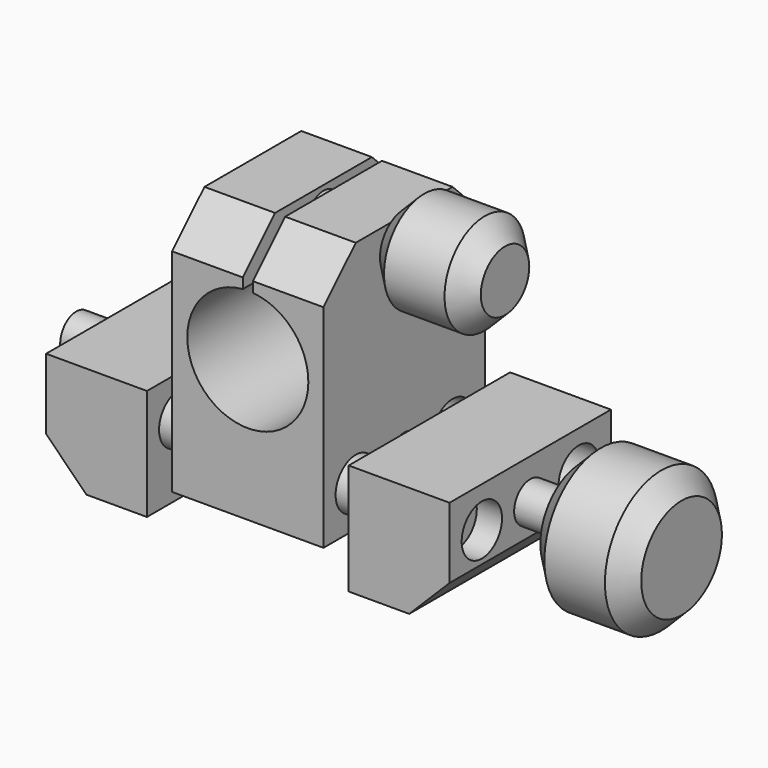
from build123d import *

# Parameters (mm, degrees)
F1_DEPTH      = 20
F2_R          = 2.5
F2_R_2        = 2
F3_DEPTH      = 7.501
F3_DEPTH_BACK = 7.501
F4_DEPTH      = 17.5
F5_START      = 10
F2_W          = 20
F2_H          = 11
F5_DEPTH      = 10
F6_START      = -10
F6_DEPTH      = 10
F7_D          = 3.3
F8_SIZE       = 4
F8_2_SIZE     = 4
F9_SIZE       = 4
F10_DEPTH     = 25
F11_R         = 7
F12_DEPTH     = 10
F14_D         = 3.3
F14_DEPTH     = 7.501
F15_D         = 4.2
F15_DEPTH     = 7.501
F16_SIZE      = 0.5
F17_R         = 2
F18_DEPTH     = 15
F19_R         = 5
F20_DEPTH     = 10
F21_SIZE      = 2
F21_2_SIZE    = 2
F22_SIZE      = 1


with BuildPart() as f1:
    # F0 (on Front) → F1 (new body)
    with BuildSketch(Plane.XZ):
        with BuildLine():
            Line((-0.5, 25), (-7.5, 25))
            Line((-7.5, 25), (-7.5, 0))
            Line((-7.5, 0), (7.5, 0))
            Line((7.5, 0), (7.5, 25))
            Line((7.5, 25), (0.5, 25))
            Line((0.5, 25), (0.5, 19.9791303716))
            ThreePointArc((0.5, 19.9791303716), (0, 8), (-0.5, 19.9791303716))
            Line((-0.5, 19.9791303716), (-0.5, 25))
        make_face()
    extrude(amount=-F1_DEPTH)

    # F2 (on Right) → F3 (cut, two sides)
    with BuildSketch(Plane.YZ) as f3_sk:
        with Locations((4, 4)):
            Circle(F2_R)
        with Locations((10, 4)):
            Circle(F2_R_2)
        with Locations((16, 4)):
            Circle(F2_R)
    extrude(amount=F3_DEPTH, mode=Mode.SUBTRACT)
    extrude(f3_sk.sketch, amount=-F3_DEPTH_BACK, mode=Mode.SUBTRACT)

    # F9
    f9_edges = [f1.edges().sort_by_distance(p)[0] for p in [
        (4, 0, 25),
        (-4, 0, 25),
        (-4, 20, 25),
        (4, 20, 25),
    ]]
    chamfer(f9_edges, length=F9_SIZE)

    # F14 (through all, one way)
    with BuildSketch(Plane.YZ):
        with Locations((10, 22.5)):
            Circle(F14_D / 2)
    extrude(amount=-F14_DEPTH, mode=Mode.SUBTRACT)

    # F15 (through all, one way)
    with BuildSketch(Plane(origin=(0, 0, 0), x_dir=(0, 1, 0), z_dir=(-1, 0, 0))):
        with Locations((10, -22.5)):
            Circle(F15_D / 2)
    extrude(amount=-F15_DEPTH, mode=Mode.SUBTRACT)


with BuildPart() as f4:
    # F2 (on Right) → F4 (new body, symmetric)
    with BuildSketch(Plane.YZ):
        with Locations((4, 4)):
            Circle(F2_R)
    extrude(amount=F4_DEPTH, both=True)

    # F16
    f16_edges = [f4.edges().sort_by_distance(p)[0] for p in [
        (-17.5, 1.5, 4),
    ]]
    chamfer(f16_edges, length=F16_SIZE)


with BuildPart() as f5:
    # F2 (on Right) → F5 (new body)
    with BuildSketch(Plane.YZ.offset(F5_START)):
        with Locations((10, 2.5)):
            Rectangle(F2_W, F2_H)
        with Locations((4, 4)):
            Circle(F2_R, mode=Mode.SUBTRACT)
        with Locations((10, 4)):
            Circle(F2_R_2, mode=Mode.SUBTRACT)
        with Locations((16, 4)):
            Circle(F2_R, mode=Mode.SUBTRACT)
    extrude(amount=F5_DEPTH)

    # F8
    f8_edges = [f5.edges().sort_by_distance(p)[0] for p in [
        (20, 10, -3),
    ]]
    chamfer(f8_edges, length=F8_SIZE)


with BuildPart() as f6:
    # F2 (on Right) → F6 (new body)
    with BuildSketch(Plane.YZ.offset(F6_START)):
        with Locations((10, 2.5)):
            Rectangle(F2_W, F2_H)
        with Locations((4, 4)):
            Circle(F2_R, mode=Mode.SUBTRACT)
        with Locations((10, 4)):
            Circle(F2_R_2, mode=Mode.SUBTRACT)
        with Locations((16, 4)):
            Circle(F2_R, mode=Mode.SUBTRACT)
        with Locations((10, 4)):
            Circle(F2_R_2)
    extrude(amount=-F6_DEPTH)

    # F7 (through all)
    with Locations(Plane.YZ):
        with Locations((10, 4)):
            Hole(F7_D / 2)

    # F8#2
    f8_2_edges = [f6.edges().sort_by_distance(p)[0] for p in [
        (-20, 10, -3),
    ]]
    chamfer(f8_2_edges, length=F8_2_SIZE)


with BuildPart() as f10:
    # F2 (on Right) → F10 (new body, symmetric)
    with BuildSketch(Plane.YZ):
        with Locations((10, 4)):
            Circle(F2_R_2)
    extrude(amount=F10_DEPTH, both=True)

    # F11 (on face) → F12 (join)
    with BuildSketch(Plane.YZ.offset(25)):
        with Locations((10, 4)):
            Circle(F11_R)
    extrude(amount=F12_DEPTH)

    # F21
    f21_edges = [f10.edges().sort_by_distance(p)[0] for p in [
        (30, 17, 4),
        (25, 3, 4),
        (35, 3, 4),
    ]]
    chamfer(f21_edges, length=F21_SIZE)


with BuildPart() as f18:
    # F17 (on face) → F18 (new body, through all)
    with BuildSketch(Plane(origin=(-7.5, 0, 0), x_dir=(0, -1, 0), z_dir=(-1, 0, 0))):
        with Locations((-10, 22.5)):
            Circle(F17_R)
    extrude(amount=-F18_DEPTH)

    # F19 (on face) → F20 (join)
    with BuildSketch(Plane.YZ.offset(7.5)):
        with Locations((10, 22.5)):
            Circle(F19_R)
    extrude(amount=F20_DEPTH)

    # F21#2
    f21_2_edges = [f18.edges().sort_by_distance(p)[0] for p in [
        (12.5, 15, 22.5),
        (7.5, 5, 22.5),
        (17.5, 5, 22.5),
    ]]
    chamfer(f21_2_edges, length=F21_2_SIZE)

    # F22
    f22_edges = [f18.edges().sort_by_distance(p)[0] for p in [
        (-7.5, 12, 22.5),
    ]]
    chamfer(f22_edges, length=F22_SIZE)


solid = Compound([f1.part, f4.part, f5.part, f6.part, f10.part, f18.part])
